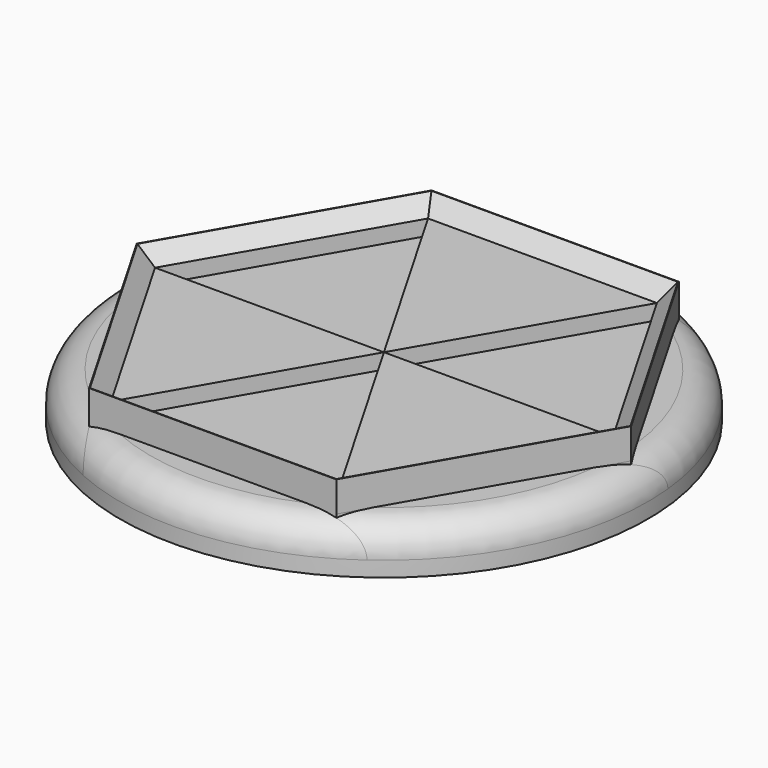
from build123d import *

# Parameters (mm, degrees)
F1_DEPTH = 12.7
F2_DEPTH = 10.16
F3_DEPTH = 7.62
F4_DEPTH = 7.62
F5_DEPTH = 10.16
F6_DEPTH = 7.62
F7_DEPTH = 10.16
F8_DEPTH = 7.62
F10_SIZE = 2.54
F11_SIZE = 2.53999
F12_SIZE = 2.53999


# Not quite as in the source:
# - a fillet or chamfer that OpenCascade refuses, or shapes differently, is made with other operations: its cross-section is extruded or revolved along the edge and cut away or added
# - a fillet or chamfer is up to 0.001 mm smaller than in the source, because OpenCascade refuses the exact size


with BuildPart() as f1:
    # F0 (on Top) → F1 (new body)
    with BuildSketch(Plane.XY):
        Polygon((-20.574, 35.6352133149), (-41.148, 0), (-20.574, -35.6352133149), (20.574, -35.6352133149), (41.148, 0), (20.574, 35.6352133149), align=None)
        Polygon((38.1, 0), (19.05, -32.9955678842), (-19.05, -32.9955678842), (-38.1, 0), (-19.05, 32.9955678842), (19.05, 32.9955678842), align=None, mode=Mode.SUBTRACT)
    extrude(amount=F1_DEPTH)

    # F0 (on Top) → F2 (join)
    with BuildSketch(Plane.XY):
        Polygon((-19.05, 32.9955678842), (0, 0), (19.05, 32.9955678842), align=None)
    extrude(amount=F2_DEPTH)

    # F0 (on Top) → F3 (join)
    with BuildSketch(Plane.XY):
        Polygon((-38.1, 0), (0, 0), (-19.05, 32.9955678842), align=None)
    extrude(amount=F3_DEPTH)

    # F0 (on Top) → F4 (join)
    with BuildSketch(Plane.XY):
        Polygon((0, 0), (38.1, 0), (19.05, 32.9955678842), align=None)
    extrude(amount=F4_DEPTH)

    # F0 (on Top) → F8 (join)
    with BuildSketch(Plane.XY):
        with BuildLine():
            ThreePointArc((43.9377985476, 0), (0, 43.9377985476), (-43.9377985476, 0))
            ThreePointArc((-43.9377985476, 0), (0, -43.9377985476), (43.9377985476, 0))
        make_face()
        with BuildLine():
            ThreePointArc((-20.574, -35.6352133149), (-35.6352133149, -20.574), (-41.148, 0))
            ThreePointArc((-41.148, 0), (-35.6352133149, 20.574), (-20.574, 35.6352133149))
            ThreePointArc((-20.574, 35.6352133149), (-10.6498860679, 39.7459159001), (0, 41.148))
            ThreePointArc((0, 41.148), (10.6498860679, 39.7459159001), (20.574, 35.6352133149))
            ThreePointArc((20.574, 35.6352133149), (35.6352133149, 20.574), (41.148, 0))
            ThreePointArc((41.148, 0), (35.6352133149, -20.574), (20.574, -35.6352133149))
            ThreePointArc((20.574, -35.6352133149), (0, -41.148), (-20.574, -35.6352133149))
        make_face(mode=Mode.SUBTRACT)
        with BuildLine():
            Line((-20.574, -35.6352133149), (-41.148, 0))
            ThreePointArc((-41.148, 0), (-35.6352133149, -20.574), (-20.574, -35.6352133149))
        make_face()
        with BuildLine():
            Line((20.574, -35.6352133149), (-20.574, -35.6352133149))
            ThreePointArc((-20.574, -35.6352133149), (0, -41.148), (20.574, -35.6352133149))
        make_face()
        with BuildLine():
            Line((41.148, 0), (20.574, -35.6352133149))
            ThreePointArc((20.574, -35.6352133149), (35.6352133149, -20.574), (41.148, 0))
        make_face()
        with BuildLine():
            ThreePointArc((41.148, 0), (35.6352133149, 20.574), (20.574, 35.6352133149))
            Line((20.574, 35.6352133149), (41.148, 0))
        make_face()
        with BuildLine():
            ThreePointArc((0, 41.148), (-10.6498860679, 39.7459159001), (-20.574, 35.6352133149))
            Line((-20.574, 35.6352133149), (20.574, 35.6352133149))
            ThreePointArc((20.574, 35.6352133149), (10.6498860679, 39.7459159001), (0, 41.148))
        make_face()
        with BuildLine():
            ThreePointArc((-20.574, 35.6352133149), (-35.6352133149, 20.574), (-41.148, 0))
            Line((-41.148, 0), (-20.574, 35.6352133149))
        make_face()
    extrude(amount=F8_DEPTH)

    # F9: fillet of radius 5.08 on 1 edges, made by hand


with BuildPart() as f5:
    # F0 (on Top) → F5 (new body)
    with BuildSketch(Plane.XY):
        Polygon((0, 0), (19.05, -32.9955678842), (38.1, 0), align=None)
    extrude(amount=F5_DEPTH)


with BuildPart() as f6:
    # F0 (on Top) → F6 (new body)
    with BuildSketch(Plane.XY):
        Polygon((-19.05, -32.9955678842), (19.05, -32.9955678842), (0, 0), align=None)
    extrude(amount=F6_DEPTH)


with BuildPart() as f7:
    # F0 (on Top) → F7 (new body)
    with BuildSketch(Plane.XY):
        Polygon((-38.1, 0), (-19.05, -32.9955678842), (0, 0), align=None)
    extrude(amount=F7_DEPTH)


with BuildPart() as f9_tool2:
    # F9_s3 → F9_t4 (revolve)
    with BuildSketch(Plane.XZ):
        with BuildLine():
            ThreePointArc((-38.8577985476, 7.62), (-42.449900996, 6.1321024484), (-43.9377985476, 2.54))
            Line((-43.9377985476, 2.54), (-43.9377985476, 7.62))
            Line((-43.9377985476, 7.62), (-38.8577985476, 7.62))
        make_face()
    revolve(axis=Axis((0, 0, 7.62), (0, 0, 1)))

    split(bisect_by=Plane(origin=(-30.861, -17.8176066575, 0), x_dir=(0, 0, 1), z_dir=(-0.8660254038, -0.5, 0)), keep=Keep.TOP)


with BuildPart() as f1_1:
    add(f1.part)

    # F9_t1: cut F9_tool2
    add(f9_tool2.part, mode=Mode.SUBTRACT)


with BuildPart() as f9_tool7:
    # F9_s8 → F9_t9 (revolve)
    with BuildSketch(Plane.XZ):
        with BuildLine():
            ThreePointArc((-38.8577985476, 7.62), (-42.449900996, 6.1321024484), (-43.9377985476, 2.54))
            Line((-43.9377985476, 2.54), (-43.9377985476, 7.62))
            Line((-43.9377985476, 7.62), (-38.8577985476, 7.62))
        make_face()
    revolve(axis=Axis((0, 0, 7.62), (0, 0, 1)))

    split(bisect_by=Plane(origin=(-30.861, 17.8176066575, 0), x_dir=(0, 0, 1), z_dir=(-0.8660254038, 0.5, 0)), keep=Keep.TOP)


with BuildPart() as f1_2:
    add(f1_1.part)

    # F9_t6: cut F9_tool7
    add(f9_tool7.part, mode=Mode.SUBTRACT)


with BuildPart() as f9_tool12:
    # F9_s13 → F9_t14 (revolve)
    with BuildSketch(Plane.XZ):
        with BuildLine():
            ThreePointArc((-38.8577985476, 7.62), (-42.449900996, 6.1321024484), (-43.9377985476, 2.54))
            Line((-43.9377985476, 2.54), (-43.9377985476, 7.62))
            Line((-43.9377985476, 7.62), (-38.8577985476, 7.62))
        make_face()
    revolve(axis=Axis((0, 0, 7.62), (0, 0, 1)))

    split(bisect_by=Plane.XZ.offset(35.6352133149), keep=Keep.TOP)


with BuildPart() as f1_3:
    add(f1_2.part)

    # F9_t11: cut F9_tool12
    add(f9_tool12.part, mode=Mode.SUBTRACT)


with BuildPart() as f9_tool17:
    # F9_s18 → F9_t19 (revolve)
    with BuildSketch(Plane.XZ):
        with BuildLine():
            ThreePointArc((-38.8577985476, 7.62), (-42.449900996, 6.1321024484), (-43.9377985476, 2.54))
            Line((-43.9377985476, 2.54), (-43.9377985476, 7.62))
            Line((-43.9377985476, 7.62), (-38.8577985476, 7.62))
        make_face()
    revolve(axis=Axis((0, 0, 7.62), (0, 0, 1)))

    split(bisect_by=Plane.XZ.offset(-35.6352133149), keep=Keep.BOTTOM)


with BuildPart() as f1_4:
    add(f1_3.part)

    # F9_t16: cut F9_tool17
    add(f9_tool17.part, mode=Mode.SUBTRACT)


with BuildPart() as f9_tool22:
    # F9_s23 → F9_t24 (revolve)
    with BuildSketch(Plane.XZ):
        with BuildLine():
            ThreePointArc((-38.8577985476, 7.62), (-42.449900996, 6.1321024484), (-43.9377985476, 2.54))
            Line((-43.9377985476, 2.54), (-43.9377985476, 7.62))
            Line((-43.9377985476, 7.62), (-38.8577985476, 7.62))
        make_face()
    revolve(axis=Axis((0, 0, 7.62), (0, 0, 1)))

    split(bisect_by=Plane(origin=(30.861, -17.8176066575, 0), x_dir=(0, 0, 1), z_dir=(0.8660254038, -0.5, 0)), keep=Keep.TOP)


with BuildPart() as f1_5:
    add(f1_4.part)

    # F9_t21: cut F9_tool22
    add(f9_tool22.part, mode=Mode.SUBTRACT)


with BuildPart() as f9_tool27:
    # F9_s28 → F9_t29 (revolve)
    with BuildSketch(Plane.XZ):
        with BuildLine():
            ThreePointArc((-38.8577985476, 7.62), (-42.449900996, 6.1321024484), (-43.9377985476, 2.54))
            Line((-43.9377985476, 2.54), (-43.9377985476, 7.62))
            Line((-43.9377985476, 7.62), (-38.8577985476, 7.62))
        make_face()
    revolve(axis=Axis((0, 0, 7.62), (0, 0, 1)))

    split(bisect_by=Plane(origin=(30.861, 17.8176066575, 0), x_dir=(0, 0, 1), z_dir=(0.8660254038, 0.5, 0)), keep=Keep.TOP)


with BuildPart() as f1_6:
    add(f1_5.part)

    # F9_t26: cut F9_tool27
    add(f9_tool27.part, mode=Mode.SUBTRACT)

    # F10
    f10_edges = [f1_6.edges().sort_by_distance(p)[0] for p in [
        (-28.575, 16.497784, 12.7),
        (28.575, -16.497784, 12.7),
        (0, -32.995568, 12.7),
        (-28.575, -16.497784, 12.7),
    ]]
    chamfer(f10_edges, length=F10_SIZE)

    # F11 (size 2.54 in the source; OpenCascade refuses exactly that, so slightly less here)
    f11_edges = [f1_6.edges().sort_by_distance(p)[0] for p in [
        (0, 32.995568, 12.7),
    ]]
    chamfer(f11_edges, length=F11_SIZE)

    # F12 (size 2.54 in the source; OpenCascade refuses exactly that, so slightly less here)
    f12_edges = [f1_6.edges().sort_by_distance(p)[0] for p in [
        (28.575, 16.497784, 12.7),
    ]]
    chamfer(f12_edges, length=F12_SIZE)


solid = Compound([f5.part, f6.part, f7.part, f1_6.part])
